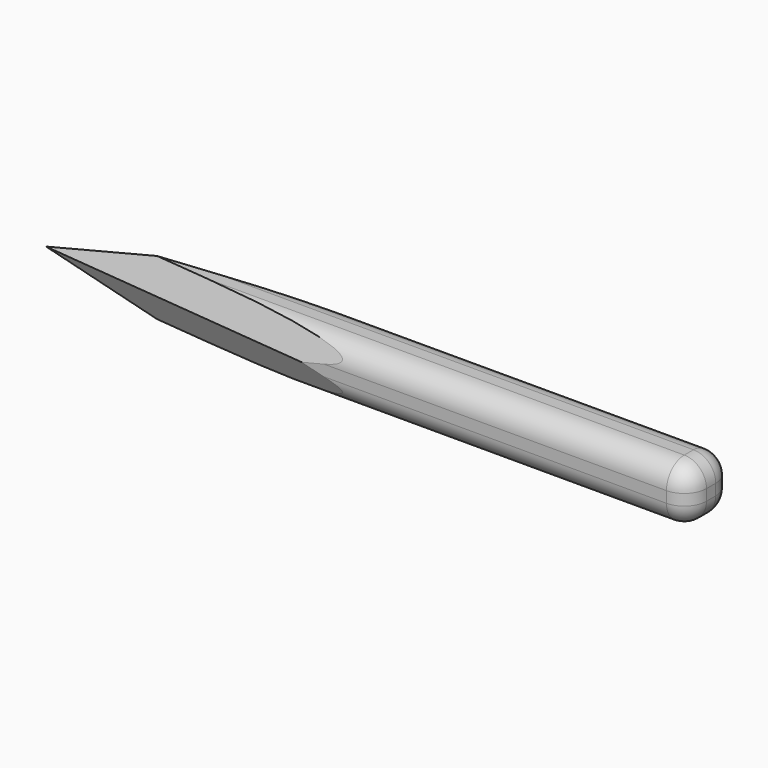
from build123d import *

# Parameters (mm, degrees)
F1_DEPTH     = 12.7
F2_SIZE2     = 6.35
F2_SIZE      = 2.54
F2_2_SIZE2   = 6.34999
F2_2_SIZE    = 2.53999
F3_T1_DEPTH  = 121.4602589597
F3_T3_DEPTH  = 121.4603587348
F3_T5_DEPTH  = 2.54
F3_T7_DEPTH  = 2.6322967076
F3_S11_W     = 5.08
F3_S11_H     = 5.08
F3_T12_DEPTH = 5.08
F3_S17_W     = 5.08
F3_S17_H     = 5.08
F3_T18_DEPTH = 5.08
F3_S23_W     = 5.08
F3_S23_H     = 5.08
F3_T24_DEPTH = 5.08
F3_S29_W     = 5.08
F3_S29_H     = 5.08
F3_T30_DEPTH = 5.08


# Not quite as in the source:
# - a fillet or chamfer that OpenCascade refuses, or shapes differently, is made with other operations: its cross-section is extruded or revolved along the edge and cut away or added
# - a fillet or chamfer is up to 0.001 mm smaller than in the source, because OpenCascade refuses the exact size


with BuildPart() as f1:
    # F0 (on Top) → F1 (new body)
    with BuildSketch(Plane.XY):
        Polygon((75.9397223592, -6.3961483538), (75.9397223592, 6.3961483538), (-12.4434158206, 6.3961483538), (-75.9397223592, 0), (-12.4434158206, -6.3961483538), align=None)
    extrude(amount=F1_DEPTH)

    # F2
    f2_edges = [f1.edges().sort_by_distance(p)[0] for p in [
        (-44.191569, -3.198074, 12.7),
        (-44.191569, 3.198074, 12.7),
    ]]
    f2_side = f1.faces().sort_by_distance((14.475683, 0, 12.7))[0]
    chamfer(f2_edges, length=F2_SIZE, length2=F2_SIZE2, reference=f2_side)

    # F2#2 (size 2.54 and 6.35 in the source; OpenCascade refuses exactly that, so slightly less here)
    f2_2_edges = [f1.edges().sort_by_distance(p)[0] for p in [
        (-44.191569, -3.198074, 0),
        (-44.191569, 3.198074, 0),
    ]]
    f2_2_side = f1.faces().sort_by_distance((14.475683, 0, 0))[0]
    chamfer(f2_2_edges, length=F2_2_SIZE, length2=F2_2_SIZE2, reference=f2_2_side)

    # F3: fillet of radius 5.08 on 8 edges, made by hand

    # F3_s2 → F3_t1 (cut)
    with BuildSketch(Plane.YZ.offset(-50.6005366005)):
        with BuildLine():
            ThreePointArc((-6.3961483538, 7.62), (-4.9082508022, 11.2121024484), (-1.3161483538, 12.7))
            Line((-1.3161483538, 12.7), (-6.3961483538, 12.7))
            Line((-6.3961483538, 12.7), (-6.3961483538, 7.62))
        make_face()
        with BuildLine():
            ThreePointArc((1.3161483538, 12.7), (4.9082508022, 11.2121024484), (6.3961483538, 7.62))
            Line((6.3961483538, 7.62), (6.3961483538, 12.7))
            Line((6.3961483538, 12.7), (1.3161483538, 12.7))
        make_face()
    extrude(amount=F3_T1_DEPTH, mode=Mode.SUBTRACT)

    # F3_s4 → F3_t3 (cut)
    with BuildSketch(Plane.YZ.offset(-50.6006363756)):
        with BuildLine():
            ThreePointArc((-6.3961483538, 5.08), (-4.9082508022, 1.4878975516), (-1.3161483538, 0))
            Line((-1.3161483538, 0), (-6.3961483538, 0))
            Line((-6.3961483538, 0), (-6.3961483538, 5.08))
        make_face()
        with BuildLine():
            ThreePointArc((1.3161483538, 0), (4.9082508022, 1.4878975516), (6.3961483538, 5.08))
            Line((6.3961483538, 5.08), (6.3961483538, 0))
            Line((6.3961483538, 0), (1.3161483538, 0))
        make_face()
    extrude(amount=F3_T3_DEPTH, mode=Mode.SUBTRACT)

    # F3_s6 → F3_t5 (cut)
    with BuildSketch(Plane.XY.offset(5.08)):
        with BuildLine():
            ThreePointArc((70.8597223592, -6.3961483538), (74.4518248076, -4.9082508022), (75.9397223592, -1.3161483538))
            Line((75.9397223592, -1.3161483538), (75.9397223592, -6.3961483538))
            Line((75.9397223592, -6.3961483538), (70.8597223592, -6.3961483538))
        make_face()
        with BuildLine():
            ThreePointArc((75.9397223592, 1.3161483538), (74.4518248076, 4.9082508022), (70.8597223592, 6.3961483538))
            Line((70.8597223592, 6.3961483538), (75.9397223592, 6.3961483538))
            Line((75.9397223592, 6.3961483538), (75.9397223592, 1.3161483538))
        make_face()
    extrude(amount=F3_T5_DEPTH, mode=Mode.SUBTRACT)

    # F3_s8 → F3_t7 (cut)
    with BuildSketch(Plane.XZ.offset(-1.3161483538)):
        with BuildLine():
            ThreePointArc((70.8597223592, 12.7), (74.4518248076, 11.2121024484), (75.9397223592, 7.62))
            Line((75.9397223592, 7.62), (75.9397223592, 12.7))
            Line((75.9397223592, 12.7), (70.8597223592, 12.7))
        make_face()
        with BuildLine():
            ThreePointArc((70.8597223592, 0), (74.4518248076, 1.4878975516), (75.9397223592, 5.08))
            Line((75.9397223592, 5.08), (75.9397223592, 0))
            Line((75.9397223592, 0), (70.8597223592, 0))
        make_face()
    extrude(amount=F3_T7_DEPTH, mode=Mode.SUBTRACT)


with BuildPart() as f3_tool10:
    # F3_s11 → F3_t12 (new body)
    with BuildSketch(Plane.XZ.offset(1.3161483538)):
        with Locations((73.3997223592, 10.16)):
            Rectangle(F3_S11_W, F3_S11_H)
    extrude(amount=F3_T12_DEPTH)

    # F3_s13 → F3_t14 (revolve, cut)
    with BuildSketch(Plane(origin=(70.8597223592, -1.3161483538, 7.62), x_dir=(-0.7071067812, 0, -0.7071067812), z_dir=(-0.7071067812, 0, 0.7071067812))):
        with BuildLine():
            ThreePointArc((0, -5.08), (5.08, 0), (0, 5.08))
            Line((0, 5.08), (0, -5.08))
        make_face()
    revolve(axis=Axis((70.8597223592, -1.3161483538, 7.62), (0, -1, 0)), mode=Mode.SUBTRACT)


with BuildPart() as f1_1:
    add(f1.part)

    # F3_t9: cut F3_tool10
    add(f3_tool10.part, mode=Mode.SUBTRACT)


with BuildPart() as f3_tool16:
    # F3_s17 → F3_t18 (new body)
    with BuildSketch(Plane.XZ.offset(1.3161483538)):
        with Locations((73.3997223592, 2.54)):
            Rectangle(F3_S17_W, F3_S17_H)
    extrude(amount=F3_T18_DEPTH)

    # F3_s19 → F3_t20 (revolve, cut)
    with BuildSketch(Plane(origin=(70.8597223592, -1.3161483538, 5.08), x_dir=(-0.7071067812, 0, 0.7071067812), z_dir=(0.7071067812, 0, 0.7071067812))):
        with BuildLine():
            ThreePointArc((0, -5.08), (5.08, 0), (0, 5.08))
            Line((0, 5.08), (0, -5.08))
        make_face()
    revolve(axis=Axis((70.8597223592, -1.3161483538, 5.08), (0, -1, 0)), mode=Mode.SUBTRACT)


with BuildPart() as f1_2:
    add(f1_1.part)

    # F3_t15: cut F3_tool16
    add(f3_tool16.part, mode=Mode.SUBTRACT)


with BuildPart() as f3_tool22:
    # F3_s23 → F3_t24 (new body)
    with BuildSketch(Plane.XZ.offset(-1.3161483538)):
        with Locations((73.3997223592, 2.54)):
            Rectangle(F3_S23_W, F3_S23_H)
    extrude(amount=-F3_T24_DEPTH)

    # F3_s25 → F3_t26 (revolve, cut)
    with BuildSketch(Plane(origin=(70.8597223592, 1.3161483538, 5.08), x_dir=(-0.7071067812, 0, 0.7071067812), z_dir=(-0.7071067812, 0, -0.7071067812))):
        with BuildLine():
            ThreePointArc((0, -5.08), (5.08, 0), (0, 5.08))
            Line((0, 5.08), (0, -5.08))
        make_face()
    revolve(axis=Axis((70.8597223592, 1.3161483538, 5.08), (0, 1, 0)), mode=Mode.SUBTRACT)


with BuildPart() as f1_3:
    add(f1_2.part)

    # F3_t21: cut F3_tool22
    add(f3_tool22.part, mode=Mode.SUBTRACT)


with BuildPart() as f3_tool28:
    # F3_s29 → F3_t30 (new body)
    with BuildSketch(Plane.XZ.offset(-1.3161483538)):
        with Locations((73.3997223592, 10.16)):
            Rectangle(F3_S29_W, F3_S29_H)
    extrude(amount=-F3_T30_DEPTH)

    # F3_s31 → F3_t32 (revolve, cut)
    with BuildSketch(Plane(origin=(70.8597223592, 1.3161483538, 7.62), x_dir=(-0.7071067812, 0, -0.7071067812), z_dir=(0.7071067812, 0, -0.7071067812))):
        with BuildLine():
            ThreePointArc((0, -5.08), (5.08, 0), (0, 5.08))
            Line((0, 5.08), (0, -5.08))
        make_face()
    revolve(axis=Axis((70.8597223592, 1.3161483538, 7.62), (0, 1, 0)), mode=Mode.SUBTRACT)


with BuildPart() as f1_4:
    add(f1_3.part)

    # F3_t27: cut F3_tool28
    add(f3_tool28.part, mode=Mode.SUBTRACT)


solid = f1_4.part
